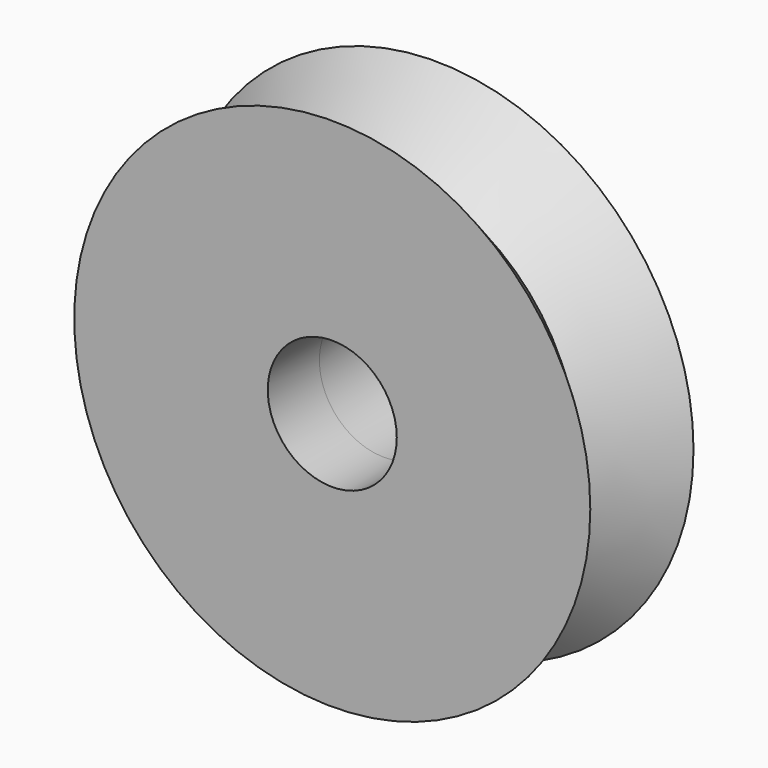
from build123d import *

# Parameters (mm, degrees)
F0_R     = 10
F0_R_2   = 2.5
F1_DEPTH = 2.5
F2_SIZE  = 2.49999


# Not quite as in the source:
# - a fillet or chamfer is up to 0.001 mm smaller than in the source, because OpenCascade refuses the exact size


with BuildPart() as f1:
    # F0 (on Front) → F1 (new body)
    with BuildSketch(Plane.XZ):
        Circle(F0_R)
        Circle(F0_R_2, mode=Mode.SUBTRACT)
    extrude(amount=F1_DEPTH)

    # F2 (size 2.5 in the source; OpenCascade refuses exactly that, so slightly less here)
    f2_edges = [f1.edges().sort_by_distance(p)[0] for p in [
        (-10, 0, 0),
    ]]
    chamfer(f2_edges, length=F2_SIZE)

    # F3: F1 across plane


with BuildPart() as f1_1:
    add(f1.part)
    add(f1.part.mirror(Plane.XZ))


solid = f1_1.part
